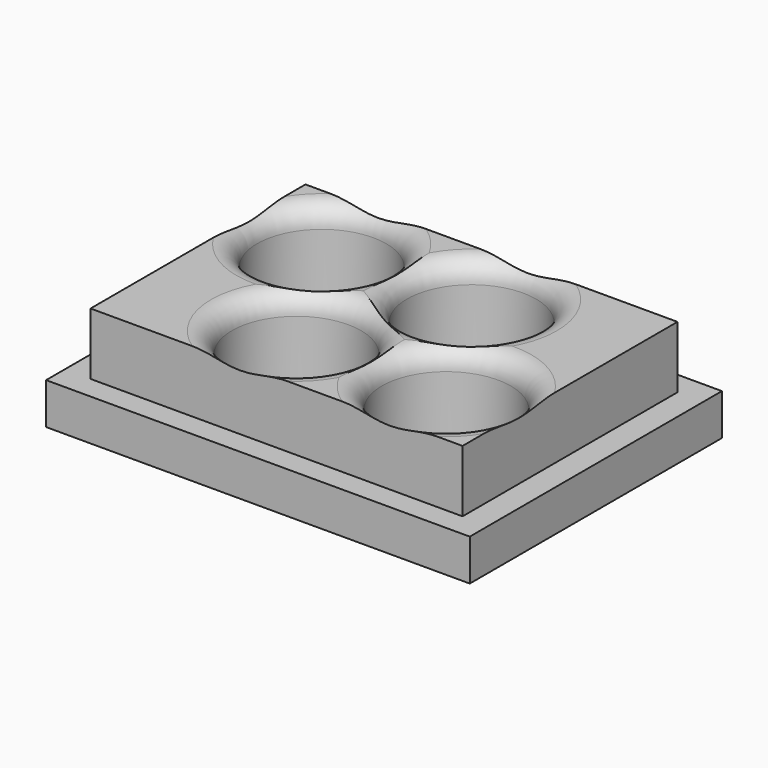
from build123d import *

# Parameters (mm, degrees)
F0_W     = 20.5
F0_H     = 15.25
F0_W_2   = 18
F0_H_2   = 13
F0_R     = 3.125
F1_DEPTH = 2
F2_DEPTH = 5


# Not quite as in the source:
# - a fillet or chamfer that OpenCascade refuses, or shapes differently, is made with other operations: its cross-section is extruded or revolved along the edge and cut away or added


with BuildPart() as f1:
    # F0 (on Top) → F1 (new body)
    with BuildSketch(Plane.XY):
        Rectangle(F0_W, F0_H)
        Rectangle(F0_W_2, F0_H_2, mode=Mode.SUBTRACT)
        Rectangle(F0_W_2, F0_H_2)
        with Locations((-1.775, -3.075)):
            Circle(F0_R, mode=Mode.SUBTRACT)
        with Locations((5.475, -3.075)):
            Circle(F0_R, mode=Mode.SUBTRACT)
        with Locations((-5.475, 3.075)):
            Circle(F0_R, mode=Mode.SUBTRACT)
        with Locations((1.775, 3.075)):
            Circle(F0_R, mode=Mode.SUBTRACT)
    extrude(amount=F1_DEPTH)

    # F0 (on Top) → F2 (join)
    with BuildSketch(Plane.XY):
        Rectangle(F0_W_2, F0_H_2)
        with Locations((-1.775, -3.075)):
            Circle(F0_R, mode=Mode.SUBTRACT)
        with Locations((5.475, -3.075)):
            Circle(F0_R, mode=Mode.SUBTRACT)
        with Locations((-5.475, 3.075)):
            Circle(F0_R, mode=Mode.SUBTRACT)
        with Locations((1.775, 3.075)):
            Circle(F0_R, mode=Mode.SUBTRACT)
    extrude(amount=F2_DEPTH)

    # F3: fillet of radius 1 on 4 edges, made by hand

    # F3_s1 → F3_t2 (revolve, cut)
    with BuildSketch(Plane.XZ.offset(-3.075)):
        with BuildLine():
            ThreePointArc((-1.35, 5), (-2.0571067812, 4.7071067812), (-2.35, 4))
            Line((-2.35, 4), (-2.35, 5))
            Line((-2.35, 5), (-1.35, 5))
        make_face()
    revolve(axis=Axis((-5.475, 3.075, 5), (0, 0, 1)), mode=Mode.SUBTRACT)

    # F3_s3 → F3_t4 (revolve, cut)
    with BuildSketch(Plane.XZ.offset(-3.075)):
        with BuildLine():
            ThreePointArc((5.9, 5), (5.1928932188, 4.7071067812), (4.9, 4))
            Line((4.9, 4), (4.9, 5))
            Line((4.9, 5), (5.9, 5))
        make_face()
    revolve(axis=Axis((1.775, 3.075, 5), (0, 0, 1)), mode=Mode.SUBTRACT)

    # F3_s5 → F3_t6 (revolve, cut)
    with BuildSketch(Plane.XZ.offset(3.075)):
        with BuildLine():
            ThreePointArc((2.35, 5), (1.6428932188, 4.7071067812), (1.35, 4))
            Line((1.35, 4), (1.35, 5))
            Line((1.35, 5), (2.35, 5))
        make_face()
    revolve(axis=Axis((-1.775, -3.075, 5), (0, 0, 1)), mode=Mode.SUBTRACT)

    # F3_s7 → F3_t8 (revolve, cut)
    with BuildSketch(Plane.XZ.offset(3.075)):
        with BuildLine():
            ThreePointArc((9.6, 5), (8.8928932188, 4.7071067812), (8.6, 4))
            Line((8.6, 4), (8.6, 5))
            Line((8.6, 5), (9.6, 5))
        make_face()
    revolve(axis=Axis((5.475, -3.075, 5), (0, 0, 1)), mode=Mode.SUBTRACT)


solid = f1.part
